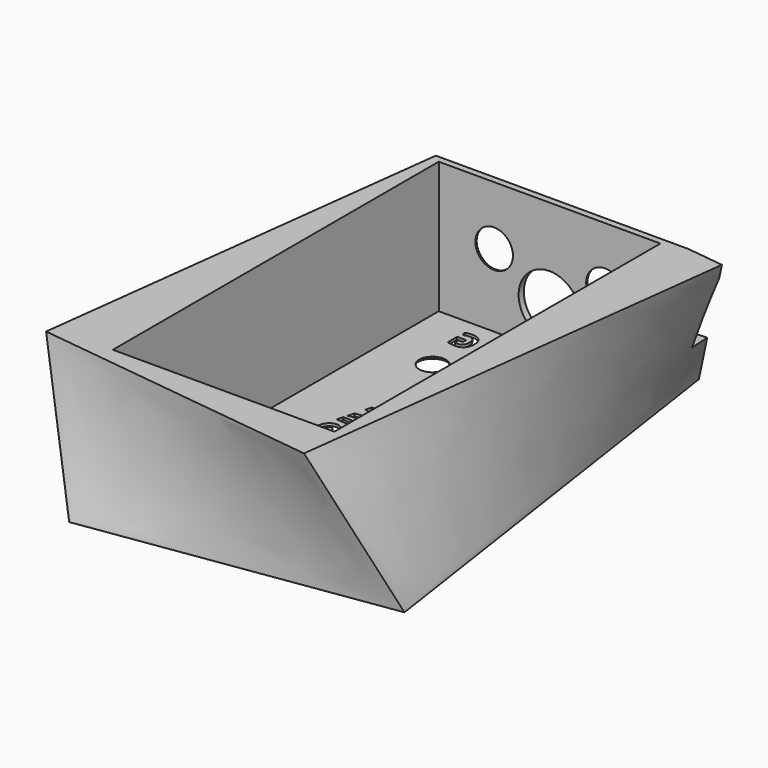
from build123d import *

# Parameters (mm, degrees)
F0_W          = 73
F0_H          = 128
F1_DEPTH      = 41.2
F5_W          = 68
F5_H          = 125
F6_DEPTH      = 40.4
F7_R          = 4.071875
F7_R_2        = 6.35
F7_R_3        = 3.675
F8_DEPTH      = 25
F10_R         = 9.5
F10_R_2       = 5.7625
F11_DEPTH     = 15
F12_W         = 68
F12_H         = 40.4
F13_DEPTH     = 25
F15_TEXT_SIZE = 9.7222222222
F16_DEPTH     = 41.2010001
F17_W         = 150
F17_H         = 29.5408671558
F18_DEPTH     = 15
F19_SIZE      = 1.5
F20_SIZE      = 0.4
F21_TEXT_SIZE = 13.8888888889
F22_DEPTH     = 41.2010001


# Not quite as in the source:
# - Text() gives the source's letters only with a copy of the font that has no kerning and outlines rounded to 1/6400 em; it was checked with that copy


with BuildPart() as f1:
    # F0 (on Top) → F1 (new body)
    with BuildSketch(Plane.XY):
        Rectangle(F0_W, F0_H)
    extrude(amount=F1_DEPTH)

    # F2 (on face) → F4 section 0
    with BuildSketch(Plane(origin=(0, 0, 0), x_dir=(1, 0, 0), z_dir=(0, 0, -1))):
        Polygon((-56.2368597455, -61.4473026316), (35.7633158502, -75.047585362), (56.2368597455, 63.4473026316), (-35.7633158502, 77.047585362), align=None)
    # F3 (on face) → F4 section 1
    with BuildSketch(Plane.XY.offset(41.2)):
        Polygon((52.4138365361, 63.0900778778), (-35.3521284594, 73.866383352), (-52.4138365361, -65.0900778778), (35.3521284594, -75.866383352), align=None)
    loft()

    # F5 (on face) → F6 (cut)
    with BuildSketch(Plane.XY.offset(41.2)):
        Rectangle(F5_W, F5_H)
    extrude(amount=-F6_DEPTH, mode=Mode.SUBTRACT)

    # F7 (on face) → F8 (cut)
    with BuildSketch(Plane.XY.offset(0.8)):
        with Locations((-17.9119046929, 40)):
            Circle(F7_R)
        with Locations((0, 40)):
            Circle(F7_R)
        with Locations((17.9119046929, 40)):
            Circle(F7_R)
        with Locations((0, -33)):
            Circle(F7_R_2)
        with Locations((8.9559523465, 15)):
            Circle(F7_R_3)
        Circle(F7_R_3)
    extrude(amount=-F8_DEPTH, mode=Mode.SUBTRACT)

    # F10 (on offset) → F11 (cut, symmetric)
    with BuildSketch(Plane.XZ.offset(-64.5)):
        with Locations((0, 13.2)):
            Circle(F10_R)
        with Locations((17, 23.2)):
            Circle(F10_R_2)
        with Locations((-17, 23.2)):
            Circle(F10_R_2)
    extrude(amount=F11_DEPTH, both=True, mode=Mode.SUBTRACT)

    # F12 (on offset) → F13 (cut)
    with BuildSketch(Plane.XZ.offset(-64.5)):
        with Locations((0, 21)):
            Rectangle(F12_W, F12_H)
    extrude(amount=-F13_DEPTH, mode=Mode.SUBTRACT)

    # F15 (on face) → F16 (cut, through all)
    with BuildSketch(Plane(origin=(0, 0, 0), x_dir=(1, 0, 0), z_dir=(0, 0, -1))):
        with Locations(Location((22.9483506944, -51), (0, 0, 180))):
            Text('V', F15_TEXT_SIZE, font='Open Sans', font_style=FontStyle.BOLD, text_align=(TextAlign.LEFT, TextAlign.BOTTOM))
        with Locations(Location((3.0328776042, -51), (0, 0, 180))):
            Text('T', F15_TEXT_SIZE, font='Open Sans', font_style=FontStyle.BOLD, text_align=(TextAlign.LEFT, TextAlign.BOTTOM))
        with Locations(Location((-16, -51), (0, 0, 180))):
            Text('G', F15_TEXT_SIZE, font='Open Sans', font_style=FontStyle.BOLD, text_align=(TextAlign.LEFT, TextAlign.BOTTOM))
    extrude(amount=-F16_DEPTH, mode=Mode.SUBTRACT)

    # F17 (on face) → F18 (cut)
    with BuildSketch(Plane(origin=(0, 64.5, 0), x_dir=(-1, 0, 0), z_dir=(0, 1, 0))):
        with Locations((0, 29.7329335779)):
            Rectangle(F17_W, F17_H)
    extrude(amount=F18_DEPTH, mode=Mode.SUBTRACT)

    # F19
    f19_edges = [f1.edges().sort_by_distance(p)[0] for p in [
        (-22.7625, 64.5, 23.2),
        (11.2375, 64.5, 23.2),
    ]]
    chamfer(f19_edges, length=F19_SIZE)

    # F20
    f20_edges = [f1.edges().sort_by_distance(p)[0] for p in [
        (13.84003, 40, 0),
        (-4.071875, 40, 0),
        (-21.98378, 40, 0),
        (5.280952, 15, 0),
        (-3.675, 0, 0),
        (-6.35, -33, 0),
    ]]
    chamfer(f20_edges, length=F20_SIZE)

    # F21 (on face) → F22 (cut, through all)
    with BuildSketch(Plane(origin=(0, 0, 0), x_dir=(1, 0, 0), z_dir=(0, 0, -1))):
        with Locations(Location((-2.1498018029, -24.3021727938), (0, 0, 105))):
            Text('TWISTED', F21_TEXT_SIZE, font='Open Sans', font_style=FontStyle.BOLDITALIC, text_align=(TextAlign.LEFT, TextAlign.BOTTOM))
        with Locations(Location((34.3407294125, -14.5245644233), (0, 0, 105))):
            Text('SCREAMER', F21_TEXT_SIZE, font='Open Sans', font_style=FontStyle.BOLDITALIC, text_align=(TextAlign.LEFT, TextAlign.BOTTOM))
    extrude(amount=-F22_DEPTH, mode=Mode.SUBTRACT)


solid = f1.part
